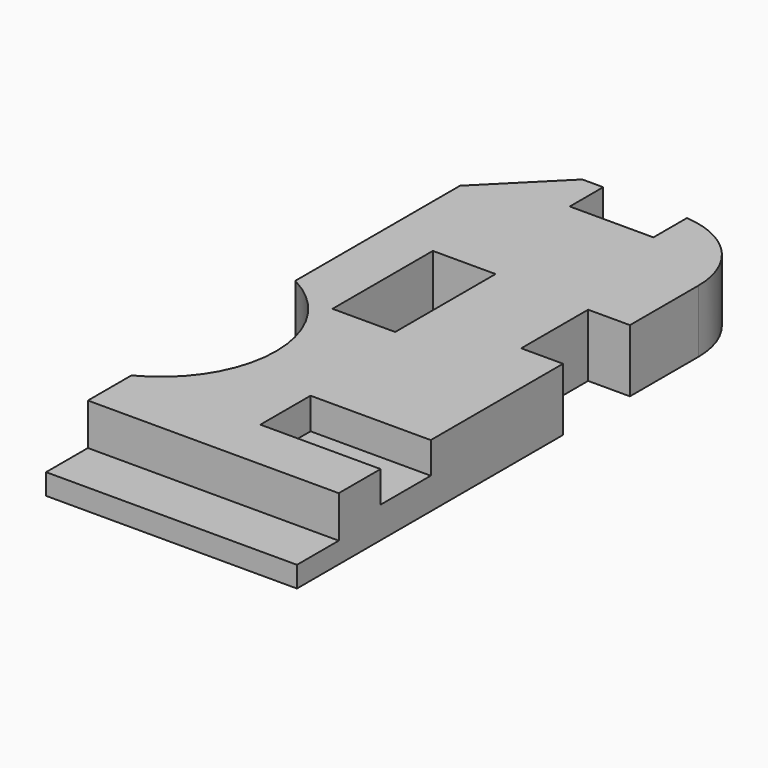
from build123d import *

# Parameters (mm, degrees)
F1_DEPTH    = 19.05
F2_W        = 76.2
F2_H        = 15.875
F3_DEPTH    = 12.7
F4_W        = 36.5125
F4_H        = 19.05
F5_DEPTH    = 9.525
F6_W        = 19.05
F6_H        = 38.1
F7_DEPTH    = 25.4
F8_T1_DEPTH = 145.8017104175


# Not quite as in the source:
# - a fillet or chamfer that OpenCascade refuses, or shapes differently, is made with other operations: its cross-section is extruded or revolved along the edge and cut away or added


with BuildPart() as f1:
    # F0 (on Top) → F1 (new body)
    with BuildSketch(Plane.XY):
        with BuildLine():
            Line((-39.025861299, -56.6028431063), (-39.025861299, -72.4778431063))
            Line((-39.025861299, -72.4778431063), (37.174138701, -72.4778431063))
            Line((37.174138701, -72.4778431063), (37.174138701, 28.547687456))
            Line((37.174138701, 28.547687456), (24.474138701, 28.547687456))
            Line((24.474138701, 28.547687456), (24.474138701, 53.947687456))
            Line((24.474138701, 53.947687456), (37.174138701, 53.947687456))
            Line((37.174138701, 53.947687456), (37.174138701, 105.3221568937))
            Line((37.174138701, 105.3221568937), (13.361638701, 105.3221568937))
            Line((13.361638701, 105.3221568937), (13.361638701, 92.6221568937))
            Line((13.361638701, 92.6221568937), (-12.038361299, 92.6221568937))
            Line((-12.038361299, 92.6221568937), (-12.038361299, 105.3221568937))
            Line((-12.038361299, 105.3221568937), (-18.388361299, 105.3221568937))
            Line((-18.388361299, 105.3221568937), (-39.025861299, 84.6846568937))
            Line((-39.025861299, 84.6846568937), (-39.025861299, 22.130676627))
            ThreePointArc((-39.025861299, 22.130676627), (-19.975861299, -8.9778431063), (-39.025861299, -40.0863628397))
            Line((-39.025861299, -40.0863628397), (-39.025861299, -40.7278431063))
            Line((-39.025861299, -40.7278431063), (-39.025861299, -56.6028431063))
        make_face()
    extrude(amount=F1_DEPTH)

    # F2 (on face) → F3 (cut)
    with BuildSketch(Plane.XY.offset(19.05)):
        with Locations((-0.925861299, -64.5403431063)):
            Rectangle(F2_W, F2_H)
    extrude(amount=-F3_DEPTH, mode=Mode.SUBTRACT)

    # F4 (on face) → F5 (cut)
    with BuildSketch(Plane.XY.offset(19.05)):
        with Locations((18.917888701, -31.2028431063)):
            Rectangle(F4_W, F4_H)
    extrude(amount=-F5_DEPTH, mode=Mode.SUBTRACT)

    # F6 (on face) → F7 (cut)
    with BuildSketch(Plane.XY.offset(19.05)):
        with Locations((-13.625861299, 35.4721568937)):
            Rectangle(F6_W, F6_H)
    extrude(amount=-F7_DEPTH, mode=Mode.SUBTRACT)

    # F8: fillet of radius 25.4 on 1 edges, made by hand

    # F8_s2 → F8_t1 (cut)
    with BuildSketch(Plane.XY.offset(-63.3758552087)):
        with BuildLine():
            ThreePointArc((37.174138701, 79.9718148102), (30.2874109671, 97.3620060109), (13.361638701, 105.3221568937))
            Line((13.361638701, 105.3221568937), (37.174138701, 105.3221568937))
            Line((37.174138701, 105.3221568937), (37.174138701, 79.9718148102))
        make_face()
    extrude(amount=F8_T1_DEPTH, mode=Mode.SUBTRACT)


solid = f1.part
